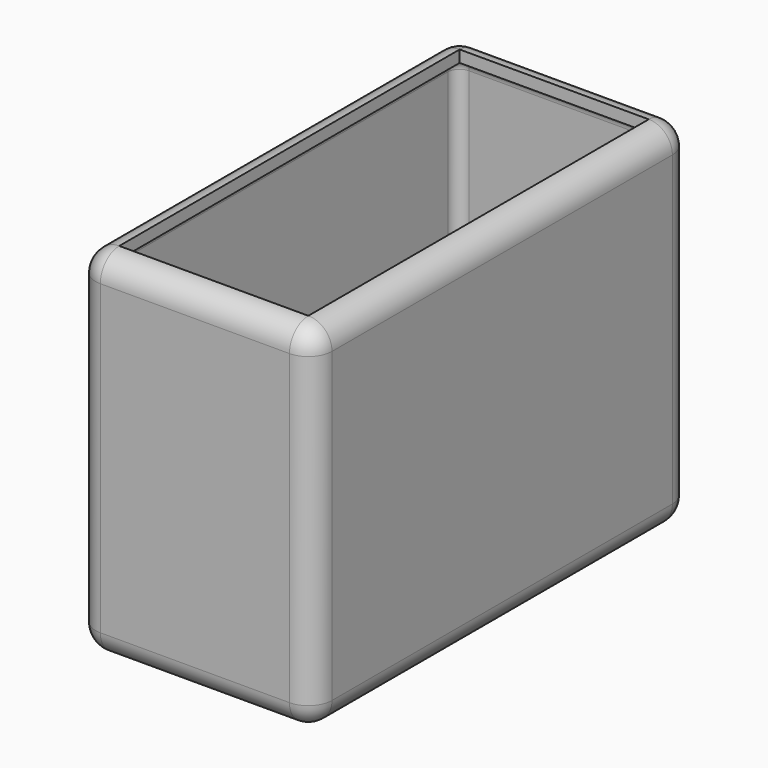
from build123d import *

# Parameters (mm, degrees)
F0_W     = 50.8
F0_H     = 101.6
F1_DEPTH = 76.2
F2_R     = 5.08
F3_T     = -2.54


# Not quite as in the source:
# - a shell that OpenCascade refuses in one call is made with other operations: the cavity is built on its own and cut out


with BuildPart() as f1:
    # F0 (on Top) → F1 (new body)
    with BuildSketch(Plane.XY):
        Rectangle(F0_W, F0_H)
    extrude(amount=F1_DEPTH)

    # F2
    f2_edges = [f1.edges().sort_by_distance(p)[0] for p in [
        (-25.4, 0, 76.2),
        (0, 50.8, 76.2),
        (-25.4, 50.8, 38.1),
        (-25.4, -50.8, 38.1),
        (0, -50.8, 76.2),
        (25.4, 0, 76.2),
        (25.4, -50.8, 38.1),
        (25.4, 50.8, 38.1),
        (0, 50.8, 0),
        (25.4, 0, 0),
        (-25.4, 0, 0),
        (0, -50.8, 0),
    ]]
    fillet(f2_edges, radius=F2_R)

    # F3: a shell. OpenCascade refuses it in one call, so the cavity is built on its own and cut out:
    # the body offset inwards by the wall thickness, plus a prism from it out through each open face.
    f3_core = offset(f1.part, amount=F3_T, mode=Mode.PRIVATE)
    f3_exits = [f3_core.faces().sort_by_distance(p)[0] for p in [
        (0, 0, 73.66),
    ]]
    add(f3_core, mode=Mode.SUBTRACT)
    extrude(f3_exits, amount=-F3_T, mode=Mode.SUBTRACT)


solid = f1.part
